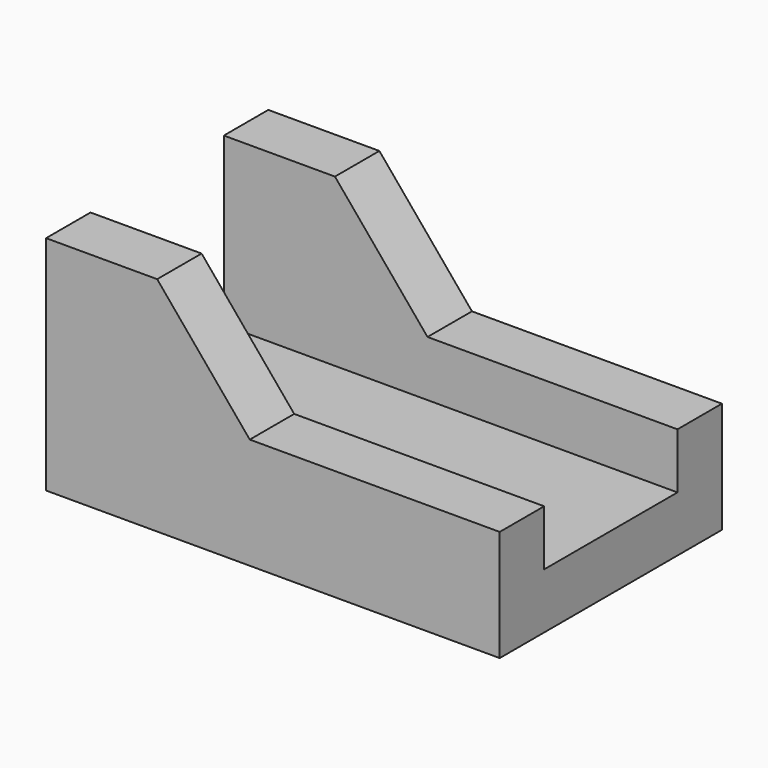
from build123d import *

# Parameters (mm, degrees)
F0_W     = 77.7875
F0_H     = 47.625
F1_DEPTH = 9.525
F3_DEPTH = 9.525


# Not quite as in the source:
# - a pattern or mirror of a feature is missing from the dataset's text; its kind, count and spacing are read off the source's solid


with BuildPart() as f1:
    # F0 (on Top) → F1 (new body)
    with BuildSketch(Plane.XY):
        Rectangle(F0_W, F0_H)
    extrude(amount=F1_DEPTH)

    # F2 (on face) → F3 (join)
    with BuildSketch(Plane.XZ.offset(23.8125)):
        Polygon((-38.89375, 38.1), (-38.89375, 0), (38.89375, 0), (38.89375, 19.05), (-3.96875, 19.05), (-19.84375, 38.1), align=None)
    f3 = extrude(amount=-F3_DEPTH)

    # F3_copies: F3 across plane
    add(f3.mirror(Plane.ZX))


solid = f1.part
